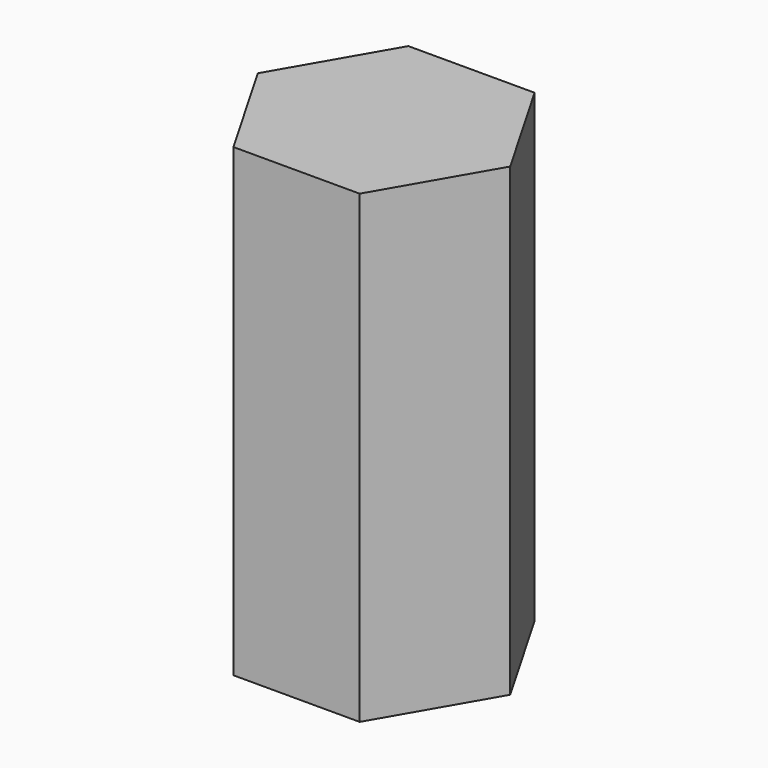
from build123d import *

# Parameters (mm, degrees)
F1_DEPTH     = 56
F2_TEXT_SIZE = 10.0762462737
F3_DEPTH     = 0.5


# Not quite as in the source:
# - Text() gives the source's letters only with a copy of the font that has no kerning and outlines rounded to 1/6400 em; it was checked with that copy


with BuildPart() as f1:
    # F0 (on Top) → F1 (new body)
    with BuildSketch(Plane.XY):
        Polygon((7.6, -13.1635861375), (15.2, 0), (7.6, 13.1635861375), (-7.6, 13.1635861375), (-15.2, 0), (-7.6, -13.1635861375), align=None)
    extrude(amount=F1_DEPTH)


with BuildPart() as f3:
    # F2 (on face) → F3 (new body)
    with BuildSketch(Plane.XY):
        with Locations(Location((-9.2787504084, -2.2207047805), (0, 0, -9.9962759464))):
            Text('OIL', F2_TEXT_SIZE, font='Open Sans', font_style=FontStyle.BOLD, text_align=(TextAlign.LEFT, TextAlign.BOTTOM))
    extrude(amount=-F3_DEPTH)


with BuildPart() as f3_1:
    # F5: moved
    add(f3.part.moved(Location((0, 0, 1))))


with BuildPart() as f1_1:
    add(f1.part)

    # F6: cut F3
    add(f3_1.part, mode=Mode.SUBTRACT)


solid = f1_1.part
